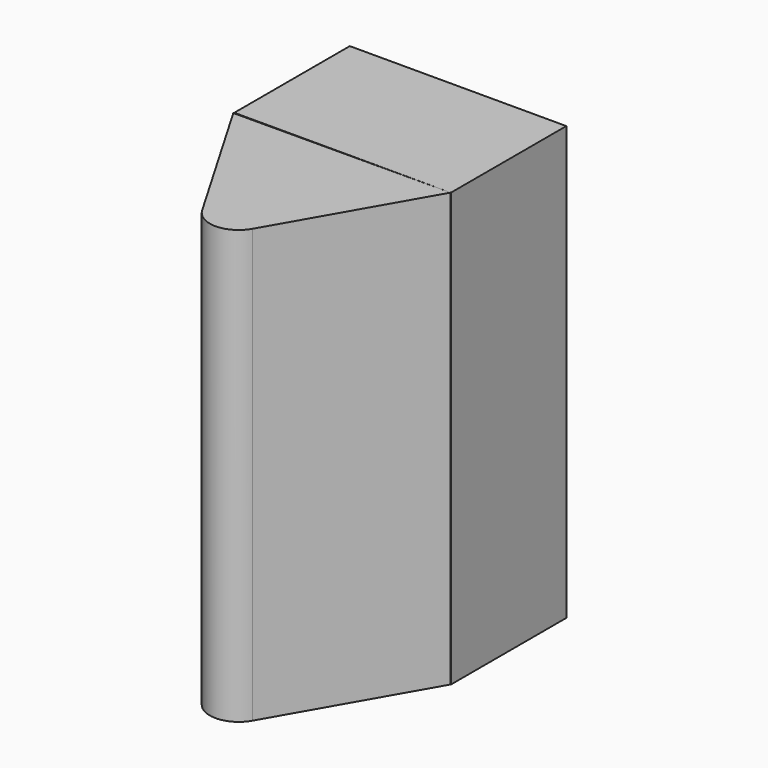
from build123d import *

# Parameters (mm, degrees)
F1_DEPTH = 76.2
F2_R     = 5.08
F3_T     = -2.54
F3_2_T   = 2.54


# Not quite as in the source:
# - a shell that OpenCascade refuses in one call is made with other operations: the cavity is built on its own and cut out


with BuildPart() as f1:
    # F0 (on Top) → F1 (new body)
    with BuildSketch(Plane.XY):
        Polygon((-18.9566183835, -33.0760292709), (-0.0466663034, 0), (-38.1463239484, -0.1615157497), align=None)
    extrude(amount=F1_DEPTH)

    # F2
    f2_edges = [f1.edges().sort_by_distance(p)[0] for p in [
        (-18.956618, -33.076029, 38.1),
    ]]
    fillet(f2_edges, radius=F2_R)

    # F3#2: shell of thickness 2.54, made by hand


with BuildPart() as f1b:
    # F0 (on Top) → F1, piece 2 (new body)
    with BuildSketch(Plane.XY):
        Polygon((-0.0466663034, 0), (0, 0), (0, 25.4), (-38.1, 25.4), (-38.1, 0), align=None)
    extrude(amount=F1_DEPTH)

    # F3
    f3_openings = [f1b.faces().sort_by_distance(p)[0] for p in [
        (-38.1, 12.7, 38.1),
    ]]
    offset(amount=F3_T, openings=f3_openings)


with BuildPart() as f3_2_core1:
    # F3_2_t2: copy of F1
    add(f1.part)

    # the walls: a layer under each face that stays
    f3_2_faces = [f3_2_core1.faces().sort_by_distance(p)[0] for p in [
        (-19.0964951259, -13.9980602828, 0),
        (-18.9781538168, -27.9960749182, 38.1),
        (-19.0964951259, -0.0807578749, 38.1),
        (-19.0964951259, -13.9980602828, 76.2),
        (-7.3181091587, -12.7187237548, 38.1),
    ]]
    thicken(f3_2_faces, amount=-F3_2_T, mode=Mode.SUBTRACT)


with BuildPart() as f1_1:
    add(f1.part)

    # what is left inside the walls is the cavity
    f3_2_cavity = [f3_2_core1.part.solids().sort_by_distance(p)[0] for p in [
        (-20.552076, -2.652352, 49.953333),
    ]]
    add(f3_2_cavity, mode=Mode.SUBTRACT)


solid = Compound([f1b.part, f1_1.part])
